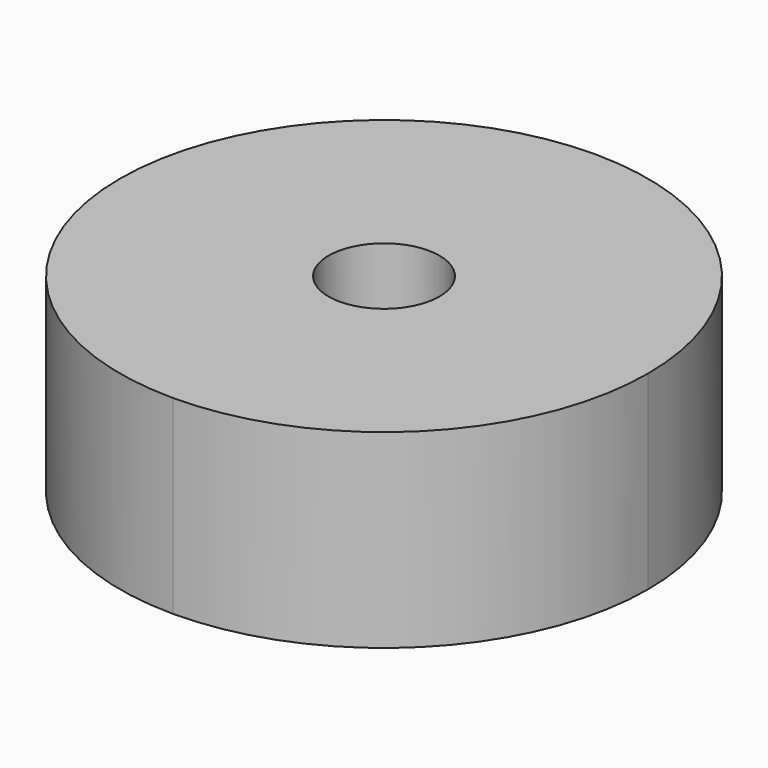
from build123d import *

# Parameters (mm, degrees)
F0_W        = 50
F0_H        = 18
F0_R        = 6.5
F1_DEPTH    = 50
F2_R        = 6.5
F3_DEPTH    = 3
F4_T1_DEPTH = 143
F5_R        = 5.25
F6_DEPTH    = 25


# Not quite as in the source:
# - a fillet or chamfer that OpenCascade refuses, or shapes differently, is made with other operations: its cross-section is extruded or revolved along the edge and cut away or added


with BuildPart() as f1:
    # F0 (on Front) → F1 (new body)
    with BuildSketch(Plane.XZ):
        Rectangle(F0_W, F0_H)
        Circle(F0_R, mode=Mode.SUBTRACT)
        Circle(F0_R)
    extrude(amount=F1_DEPTH)

    # F2 (on Front) → F3 (cut)
    with BuildSketch(Plane.XZ):
        Circle(F2_R)
    extrude(amount=F3_DEPTH, mode=Mode.SUBTRACT)

    # F4: fillet of radius 25 on 4 edges, made by hand

    # F4_s2 → F4_t1 (cut)
    with BuildSketch(Plane.XY.offset(-71.5)):
        with BuildLine():
            ThreePointArc((-25, -25), (-17.6776695297, -7.3223304703), (0, 0))
            Line((0, 0), (-25, 0))
            Line((-25, 0), (-25, -25))
        make_face()
        with BuildLine():
            ThreePointArc((25, -25), (17.6776695297, -7.3223304703), (0, 0))
            Line((0, 0), (25, 0))
            Line((25, 0), (25, -25))
        make_face()
        with BuildLine():
            ThreePointArc((25, -25), (17.6776695297, -42.6776695297), (0, -50))
            Line((0, -50), (25, -50))
            Line((25, -50), (25, -25))
        make_face()
        with BuildLine():
            ThreePointArc((-25, -25), (-17.6776695297, -42.6776695297), (0, -50))
            Line((0, -50), (-25, -50))
            Line((-25, -50), (-25, -25))
        make_face()
    extrude(amount=F4_T1_DEPTH, mode=Mode.SUBTRACT)

    # F5 (on face) → F6 (cut)
    with BuildSketch(Plane.XY.offset(9)):
        with Locations((0, -25)):
            Circle(F5_R)
    extrude(amount=-F6_DEPTH, mode=Mode.SUBTRACT)


solid = f1.part
